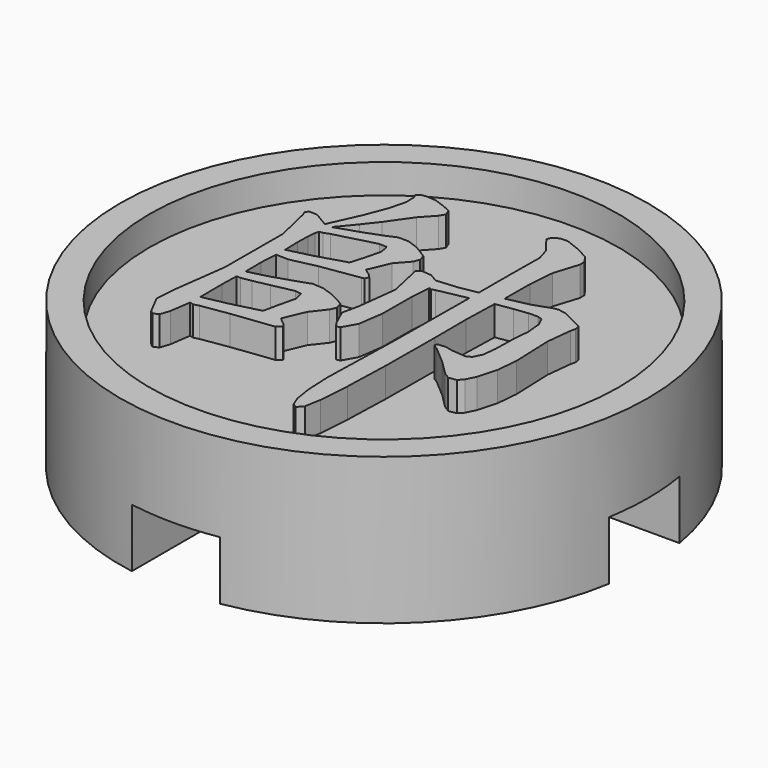
from build123d import *

# Parameters (mm, degrees)
F0_R     = 9
F1_DEPTH = 4
F3_W     = 3
F3_H     = 3
F4_DEPTH = 2
F2_R     = 9
F2_R_2   = 8
F5_DEPTH = 1
F7_DEPTH = 1


# Not quite as in the source:
# - a feature names something its author has since deleted; it is built from what else it names


with BuildPart() as f1:
    # F0 (on Top) → F1 (new body)
    with BuildSketch(Plane.XY):
        with Locations((-31.3306450844, 19.7580661625)):
            Circle(F0_R)
    extrude(amount=F1_DEPTH)

    # F3 (on face) → F4 (cut)
    with BuildSketch(Plane(origin=(0, 0, 0), x_dir=(1, 0, 0), z_dir=(0, 0, -1))):
        with BuildLine():
            ThreePointArc((-32.8306450844, -28.6321858371), (-32.0832814269, -28.7265408676), (-31.3306450844, -28.7580661625))
            ThreePointArc((-31.3306450844, -28.7580661625), (-30.5780087419, -28.7265408676), (-29.8306450844, -28.6321858371))
            Line((-29.8306450844, -28.6321858371), (-29.8306450844, -21.2580661625))
            Line((-29.8306450844, -21.2580661625), (-32.8306450844, -21.2580661625))
            Line((-32.8306450844, -21.2580661625), (-32.8306450844, -28.6321858371))
        make_face()
        with BuildLine():
            ThreePointArc((-40.204764759, -18.2580661625), (-40.2991197895, -19.0054298199), (-40.3306450844, -19.7580661625))
            ThreePointArc((-40.3306450844, -19.7580661625), (-40.2991197895, -20.510702505), (-40.204764759, -21.2580661625))
            Line((-40.204764759, -21.2580661625), (-32.8306450844, -21.2580661625))
            Line((-32.8306450844, -21.2580661625), (-32.8306450844, -18.2580661625))
            Line((-32.8306450844, -18.2580661625), (-40.204764759, -18.2580661625))
        make_face()
        with Locations((-31.3306450844, -19.7580661625)):
            Rectangle(F3_W, F3_H)
        with BuildLine():
            Line((-29.8306450844, -18.2580661625), (-29.8306450844, -21.2580661625))
            Line((-29.8306450844, -21.2580661625), (-22.4565254097, -21.2580661625))
            ThreePointArc((-22.4565254097, -21.2580661625), (-22.3621703793, -20.510702505), (-22.3306450844, -19.7580661625))
            ThreePointArc((-22.3306450844, -19.7580661625), (-22.3621703793, -19.0054298199), (-22.4565254097, -18.2580661625))
            Line((-22.4565254097, -18.2580661625), (-29.8306450844, -18.2580661625))
        make_face()
        with BuildLine():
            Line((-32.8306450844, -10.8839464878), (-32.8306450844, -18.2580661625))
            Line((-32.8306450844, -18.2580661625), (-29.8306450844, -18.2580661625))
            Line((-29.8306450844, -18.2580661625), (-29.8306450844, -10.8839464878))
            ThreePointArc((-29.8306450844, -10.8839464878), (-30.5780087419, -10.7895914574), (-31.3306450844, -10.7580661625))
            ThreePointArc((-31.3306450844, -10.7580661625), (-32.0832814269, -10.7895914574), (-32.8306450844, -10.8839464878))
        make_face()
    extrude(amount=-F4_DEPTH, mode=Mode.SUBTRACT)

    # F2 (on face) → F5 (join)
    with BuildSketch(Plane.XY.offset(4)):
        with Locations((-31.3306450844, 19.7580661625)):
            Circle(F2_R)
        with Locations((-31.3306450844, 19.7580661625)):
            Circle(F2_R_2, mode=Mode.SUBTRACT)
    extrude(amount=F5_DEPTH)

    # F6 (on face) → F7 (join)
    with BuildSketch(Plane.XY.offset(4)):
        Polygon((-35.402364897, 15.7479844977), (-35.3003342018, 16.455418297), (-35.1642871045, 16.4188721064), (-34.9840304081, 16.4690236238), (-34.0589298914, 16.6118826397), (-32.6508557007, 16.7853459281), (-32.4944160389, 16.9179685554), (-32.5853835365, 17.037016707), (-32.8379243158, 17.2478961864), (-32.5241749917, 17.9816644686), (-32.1508892513, 18.4586715435), (-32.062470053, 18.6653059143), (-32.1373086054, 18.907641156), (-32.6202514283, 19.1635570436), (-33.0428433665, 19.3123579778), (-33.4220710251, 19.3344720327), (-33.7732365403, 19.2103334527), (-34.627762124, 18.9331303192), (-35.2629180107, 18.7749938479), (-35.2688722693, 19.4433084764), (-35.2357135274, 20.0402275332), (-34.8139730791, 20.0265913554), (-33.9373396107, 20.2204595488), (-32.6270695172, 20.42111498), (-32.5394771279, 20.439008607), (-32.4808107121, 20.5674108064), (-32.5734997001, 20.6694044804), (-32.8243189891, 20.8564854359), (-32.5122664744, 21.5800666911), (-32.1373086054, 22.0026647995), (-32.0573796246, 22.2084415102), (-32.1236785978, 22.4243990776), (-32.5726482102, 22.7041566806), (-32.9654565147, 22.8452695254), (-33.3200218191, 22.8444056951), (-33.654194559, 22.6998992315), (-34.22983254, 22.4847437921), (-35.075861736, 22.2033202307), (-34.5920489126, 22.7883184298), (-34.2085761452, 23.2780484905), (-33.6567428583, 24.0611723322), (-33.2596647642, 24.4922853389), (-33.1516798102, 24.6793045923), (-33.2324541107, 24.8868089635), (-33.5376947067, 25.022862231), (-33.8650493576, 25.1384920828), (-34.1958223083, 25.1614452871), (-34.378627304, 25.1384920828), (-34.4866184281, 25.0253920196), (-34.433048611, 24.914019617), (-34.4211462639, 24.576447088), (-34.5597416605, 24.0263106106), (-34.8564858688, 23.2517016673), (-35.3139395285, 22.2407117409), (-35.3275448553, 22.2271372653), (-35.8139041269, 22.5162118948), (-35.9788574531, 22.5289842424), (-36.1063989073, 22.5264544537), (-36.1718704545, 22.4150203489), (-36.120003617, 22.2951330479), (-35.9388929627, 21.5112070782), (-35.8411129293, 21.0673217239), (-35.8470641029, 18.6253414239), (-36.0927948146, 16.7717159205), (-36.1370093499, 16.0693972304), (-35.8036998233, 15.4282870851), (-35.6906127176, 15.3381587369), (-35.5112013408, 15.4146817583), align=None)
        Polygon((-33.4841248895, 17.2852938669), (-33.5079419241, 17.2852938669), (-34.4619622442, 17.0446801155), (-35.286728875, 16.8771587453), (-35.2935346235, 17.7963173438), (-35.2765233374, 18.4076685363), (-35.1345281517, 18.4017081075), (-34.7893168951, 18.4612383535), (-34.2493921254, 18.5734684162), (-33.5215472508, 18.72397233), (-33.310686282, 18.6967616765), (-33.2324541107, 18.3940693798), (-33.3761646165, 17.7954720242), align=None, mode=Mode.SUBTRACT)
        Polygon((-33.5002970262, 20.8904833273), (-33.5079419241, 20.8836960894), (-34.4253975429, 20.6056044447), (-35.2221082006, 20.4109341233), (-35.2391133165, 20.9576769818), (-35.2272109694, 21.3810772183), (-35.2000003159, 21.6616986516), (-35.171092853, 21.7815859526), (-35.0495025723, 21.8045391569), (-34.8547890593, 21.8733987698), (-33.4705442436, 22.2407117409), (-33.2188487839, 22.2271372653), (-33.1797357833, 22.0962052773), (-33.1542219393, 21.9107902801), (-33.291965846, 21.3538665648), (-33.4297097527, 20.8972705651), align=None, mode=Mode.SUBTRACT)
        Polygon((-30.6373969166, 21.0945323774), (-29.6510693445, 21.2917941897), (-29.6740225488, 18.2529071733), (-29.7157332104, 16.509839604), (-29.7454736525, 15.3594151317), (-29.7054906514, 14.5057348677), (-29.6145416645, 13.9283939069), (-29.4911990424, 13.6086890901), (-29.3399053409, 13.5058050539), (-29.1749137594, 13.6869157082), (-29.0797073232, 14.238743442), (-29.0039987703, 15.2973427566), (-28.9546987428, 16.8627019288), (-28.9402604368, 18.9348518095), (-28.9470476747, 20.279138305), (-28.9130497833, 21.4516644917), (-28.3339749918, 21.5409475203), (-27.8791066527, 21.597898616), (-27.5627596675, 21.6072773446), (-27.3961638298, 21.5571134868), (-27.2609126904, 21.271370774), (-27.2124764931, 20.7782470944), (-27.2609126904, 20.133768011), (-27.2770786569, 19.448405075), (-27.3281063449, 18.9875454559), (-27.4641596124, 18.7103670033), (-27.6095916085, 18.6083424782), (-27.858683237, 18.628741213), (-28.1290621114, 18.6508552679), (-28.3858665102, 18.7103670033), (-28.661366664, 18.6831563498), (-28.6741390116, 18.5811318247), (-28.5185261587, 18.485882197), (-27.9164981629, 17.9731742511), (-27.4369489589, 17.4961733464), (-27.2235211801, 17.360977739), (-26.9607933738, 17.4043358483), (-26.816225208, 17.5607755101), (-26.6580825665, 17.8804914334), (-26.4778505509, 18.5216015787), (-26.4097930661, 19.2613549706), (-26.4625484147, 20.6439214874), (-26.3690079369, 21.5026921798), (-26.3281611056, 21.6659561008), (-26.3553717591, 21.8325519385), (-27.1070274981, 22.2135010875), (-27.3706191346, 22.2602713263), (-27.5559724296, 22.2271372653), (-28.1401685006, 22.023026513), (-28.8994136055, 21.859762592), (-28.8917625374, 22.9422036221), (-28.8212369661, 23.8052317637), (-28.555917669, 24.6487003199), (-28.5644325673, 24.8536132003), (-28.7429986245, 25.0840707758), (-29.1477031059, 25.3051496227), (-29.6647055223, 25.5058050539), (-29.9197822605, 25.4922305782), (-30.1136381134, 25.3731454053), (-30.1697500597, 25.2396836287), (-30.0728036226, 25.0976452515), (-29.7684268568, 24.717621635), (-29.6374948688, 24.2813873488), (-29.6494033861, 23.1369356458), (-29.6510693445, 21.6999539921), (-30.2938886396, 21.5894454198), (-30.9911107312, 21.5299028333), (-31.2734104633, 21.6974242035), (-31.6373359857, 21.7271646456), (-31.7487207288, 21.62683693), (-31.7291734838, 21.5299028333), (-31.4919286705, 20.4517192524), (-31.6509413125, 19.1185021248), (-31.7776281917, 18.5258466874), (-31.5182940043, 17.9587236047), (-31.4910833508, 17.9315129512), (-31.4137026693, 17.8099226706), (-31.2802038714, 17.8396816234), (-31.0217396845, 18.304780181), (-30.8992794033, 19.1559183159), (-30.8933374851, 20.4058128438), (-30.8482763961, 21.0809579017), (-30.7683474153, 21.0580046974), align=None)
    extrude(amount=F7_DEPTH)


solid = f1.part
